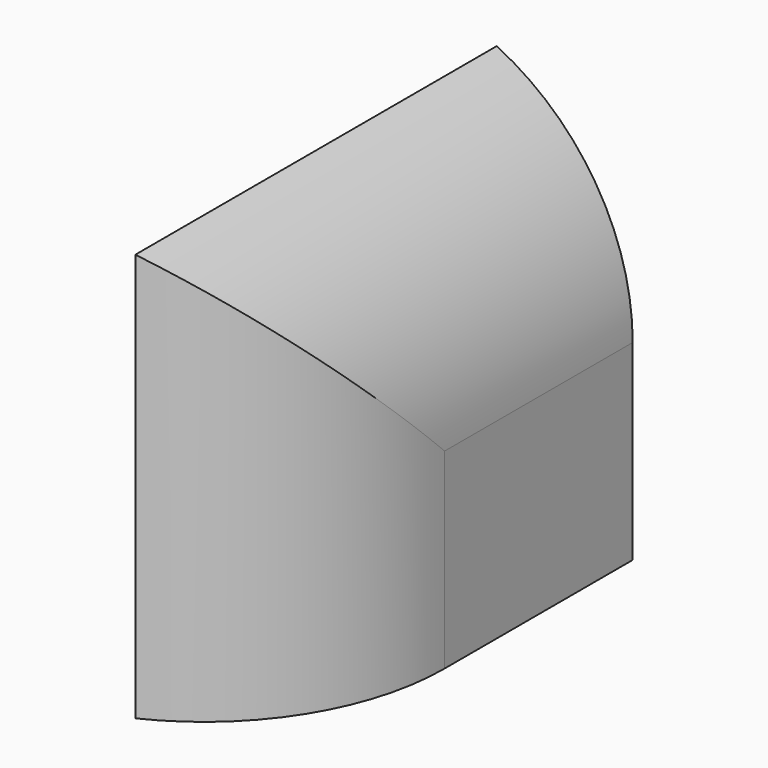
from build123d import *

# Parameters (mm, degrees)
F0_W        = 95.3594446182
F0_H        = 86.1524492502
F1_DEPTH    = 28.702
F2_T1_DEPTH = 314.8617842149
F2_T3_DEPTH = 324.0687795829


# Not quite as in the source:
# - a fillet or chamfer that OpenCascade refuses, or shapes differently, is made with other operations: its cross-section is extruded or revolved along the edge and cut away or added


with BuildPart() as f1:
    # F0 (on Right) → F1 (new body)
    with BuildSketch(Plane.YZ):
        with Locations((-228.6328673363, 162.2415110469)):
            Rectangle(F0_W, F0_H)
    extrude(amount=F1_DEPTH)

    # F2: fillet of radius 50.8 on 2 edges, made by hand

    # F2_s2 → F2_t1 (cut)
    with BuildSketch(Plane.XY.offset(4.8106189394)):
        with BuildLine():
            ThreePointArc((0, -276.3125896454), (20.9323288391, -257.5712930168), (28.702, -230.5707226524))
            Line((28.702, -230.5707226524), (28.702, -276.3125896454))
            Line((28.702, -276.3125896454), (0, -276.3125896454))
        make_face()
    extrude(amount=F2_T1_DEPTH, mode=Mode.SUBTRACT)

    # F2_s4 → F2_t3 (cut)
    with BuildSketch(Plane.XZ.offset(66.5984775448)):
        with BuildLine():
            ThreePointArc((0, 205.317735672), (20.9323288391, 186.5764390434), (28.702, 159.5758686791))
            Line((28.702, 159.5758686791), (28.702, 205.317735672))
            Line((28.702, 205.317735672), (0, 205.317735672))
        make_face()
    extrude(amount=F2_T3_DEPTH, mode=Mode.SUBTRACT)


solid = f1.part
